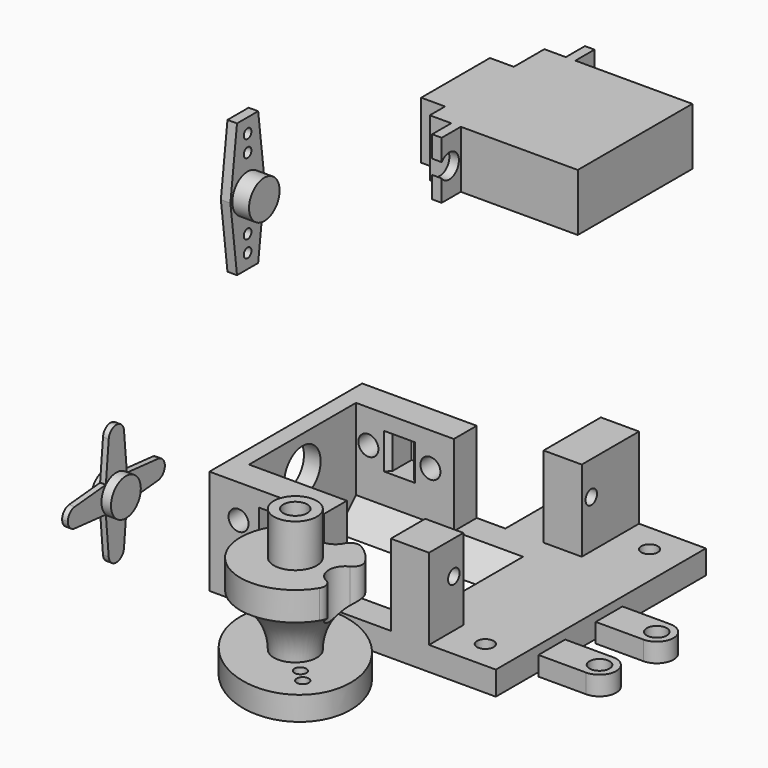
from build123d import *

# Parameters (mm, degrees)
F2_W           = 30
F2_H           = 15
F3_DEPTH       = 5
F5_DEPTH       = 17
F6_R           = 4.75
F7_DEPTH       = 14.501
F8_W           = 4.5
F8_H           = 7.5
F8_R           = 2.1
F9_DEPTH       = 55.001
F10_W          = 30
F10_H          = 12
F11_DEPTH      = 31
F12_W          = 2
F12_H          = 12
F13_DEPTH      = 5
F13_DEPTH_BACK = 35
F14_W          = 18
F14_H          = 12
F15_DEPTH      = 5
F16_R          = 2.75
F17_DEPTH      = 3
F19_DEPTH      = 1.2
F20_COUNT      = 4
F21_R          = 3.9
F22_DEPTH      = 2
F22_DEPTH_BACK = 2.2
F23_R          = 2.5
F24_DEPTH      = 55.501
F25_W          = 8
F25_H          = 9
F25_H_2        = 15
F26_DEPTH      = 17
F28_DEPTH      = 2
F29_R          = 1
F30_DEPTH      = 13.001
F31_R          = 4
F32_DEPTH      = 3.5
F37_R          = 3.5
F38_DEPTH      = 10.6200078449
F39_T1_DEPTH   = 19.8766819715
F41_DEPTH      = 5
F42_R          = 2.5
F43_DEPTH      = 31.0010001
F45_D          = 2.5
F45_DEPTH      = 6
F45_TIP        = 0.7510757738
F46_R          = 2.1
F47_DEPTH      = 4
F49_D          = 3
F49_DEPTH      = 8
F49_TIP        = 0.9012909285
F50_SIZE       = 1
F52_D          = 3.5
F53_R          = 3
F56_DEPTH      = 35


# Not quite as in the source:
# - a fillet or chamfer that OpenCascade refuses, or shapes differently, is made with other operations: its cross-section is extruded or revolved along the edge and cut away or added


with BuildPart() as f3:
    # F2 (on Top) → F3 (new body)
    with BuildSketch(Plane.XY):
        Polygon((0, 15), (0, 0), (60, 0), (60, 40), (30, 40), (0, 40), (0, 25), align=None)
        with Locations((45, 47.5)):
            Rectangle(F2_W, F2_H)
        with BuildLine():
            Line((-6, 15), (0, 15))
            Line((0, 15), (0, 25))
            Line((0, 25), (-6, 25))
            ThreePointArc((-6, 25), (-11, 20), (-6, 15))
        make_face()
    extrude(amount=F3_DEPTH)

    # F4 (on face) → F5 (join)
    with BuildSketch(Plane.XY.offset(5)):
        Polygon((0, 0), (24, 0), (24, 6), (3.5, 6), (3.5, 34), (24, 34), (24, 40), (0, 40), (0, 25), (0, 15), align=None)
    extrude(amount=F5_DEPTH)

    # F6 (on face) → F7 (cut, through all)
    with BuildSketch(Plane.YZ.offset(3.5)):
        with Locations((20, 15)):
            Circle(F6_R)
    extrude(amount=-F7_DEPTH, mode=Mode.SUBTRACT)

    # F8 (on face) → F9 (cut, through all)
    with BuildSketch(Plane.XZ):
        with Locations((12.6, 15)):
            Rectangle(F8_W, F8_H)
        with Locations((6.1, 15)):
            Circle(F8_R)
        with Locations((19.1, 15)):
            Circle(F8_R)
    extrude(amount=-F9_DEPTH, mode=Mode.SUBTRACT)

    # F25 (on face) → F26 (join)
    with BuildSketch(Plane.XY.offset(5)):
        with Locations((42, 4.5)):
            Rectangle(F25_W, F25_H)
        with Locations((42, 47.5)):
            Rectangle(F25_W, F25_H_2)
    extrude(amount=F26_DEPTH)

    # F49
    with Locations(Plane.YZ.offset(46)):
        with Locations((6.5, 15), (42.5, 15)):
            Hole(F49_D / 2, depth=F49_DEPTH)
            with Locations((0, 0, -(F49_DEPTH + F49_TIP / 2))):  # 118° drill point
                Cone(0, F49_D / 2, F49_TIP, mode=Mode.SUBTRACT)

    # F50
    f50_edges = [f3.edges().sort_by_distance(p)[0] for p in [
        (10.35, 34, 15),
        (14.85, 34, 15),
        (10.35, 6, 15),
        (14.85, 6, 15),
    ]]
    chamfer(f50_edges, length=F50_SIZE)

    # F52 (through all)
    with Locations(Plane.XY.offset(5)):
        with Locations((53, 49), (53, 6), (-6, 20)):
            Hole(F52_D / 2)

    # F53
    f53_edges = [f3.edges().sort_by_distance(p)[0] for p in [
        (0, 15, 2.5),
        (0, 25, 2.5),
    ]]
    fillet(f53_edges, radius=F53_R)

    # F55 (on face) → F56 (cut)
    with BuildSketch(Plane.YZ.offset(3.5)):
        Polygon((34, 5), (6, 5), (12, -1), (28, -1), align=None)
    extrude(amount=F56_DEPTH, mode=Mode.SUBTRACT)


with BuildPart() as f11:
    # F10 (on Right) → F11 (new body)
    with BuildSketch(Plane.YZ):
        with Locations((72.7043356746, 58.2544325833)):
            Rectangle(F10_W, F10_H)
    extrude(amount=F11_DEPTH)

    # F12 (on face) → F13 (join, two sides)
    with BuildSketch(Plane.XZ.offset(-57.7043356746)) as f13_sk:
        with Locations((5.5, 58.2544325833)):
            Rectangle(F12_W, F12_H)
    extrude(amount=F13_DEPTH)
    extrude(f13_sk.sketch, amount=-F13_DEPTH_BACK)

    # F14 (on face) → F15 (join)
    with BuildSketch(Plane(origin=(0, 0, 0), x_dir=(0, -1, 0), z_dir=(-1, 0, 0))):
        with Locations((-70.7043356746, 58.2544325833)):
            Rectangle(F14_W, F14_H)
    extrude(amount=F15_DEPTH)

    # F16 (on face) → F17 (join)
    with BuildSketch(Plane(origin=(-5, 0, 0), x_dir=(0, -1, 0), z_dir=(-1, 0, 0))):
        with Locations((-68.2043356746, 58.2544325833)):
            Circle(F16_R)
    extrude(amount=F17_DEPTH)

    # F23 (on face) → F24 (cut, through all)
    with BuildSketch(Plane(origin=(4.5, 0, 0), x_dir=(0, -1, 0), z_dir=(-1, 0, 0))):
        with BuildLine():
            ThreePointArc((-92.7043356746, 56.7544325833), (-89.9137662596, 55.8827243381), (-88.2043356746, 58.2544325833))
            ThreePointArc((-88.2043356746, 58.2544325833), (-89.9137662596, 60.6261408284), (-92.7043356746, 59.7544325833))
            Line((-92.7043356746, 59.7544325833), (-92.7043356746, 56.7544325833))
        make_face()
        with Locations((-54.7043356746, 58.2544325833)):
            Circle(F23_R)
    extrude(amount=-F24_DEPTH, mode=Mode.SUBTRACT)


with BuildPart() as f19:
    # F18 (on Right) → F19 (new body)
    with BuildSketch(Plane.YZ):
        with BuildLine():
            ThreePointArc((-25.8660980829, 41.5474520288), (-27.2194870474, 41.0230042308), (-27.8660980829, 39.7235422843))
            Line((-27.8660980829, 39.7235422843), (-28.6160980829, 31.5974520288))
            Line((-28.6160980829, 31.5974520288), (-36.7421883384, 30.8474520288))
            ThreePointArc((-36.7421883384, 30.8474520288), (-38.041650285, 30.2008409932), (-38.5660980829, 28.8474520288))
            Line((-38.5660980829, 28.8474520288), (-25.8660980829, 28.8474520288))
            Line((-25.8660980829, 28.8474520288), (-25.8660980829, 41.5474520288))
        make_face()
    extrude(amount=F19_DEPTH)

    # F20: F19 ×4 about axis
    f20_axis = Axis((0.6, -25.8660980829, 28.8474520288), (-1, 0, 0))


with BuildPart() as f19_1:
    add(f19.part)
    for i in range(1, F20_COUNT):
        add(f19.part.rotate(f20_axis, i * 360 / F20_COUNT))

    # F21 (on face) → F22 (join, two sides)
    with BuildSketch(Plane.YZ.offset(1.2)) as f22_sk:
        with Locations((-25.8660980829, 28.8474520288)):
            Circle(F21_R)
    extrude(amount=F22_DEPTH)
    extrude(f22_sk.sketch, amount=-F22_DEPTH_BACK)


with BuildPart() as f28:
    # F27 (on Right) → F28 (new body)
    with BuildSketch(Plane.YZ):
        Polygon((4.7284779331, 84.9464619864), (2.9985385872, 70.9464619864), (4.7284779331, 56.9464619864), (10.2685992414, 56.9464619864), (11.9985385872, 70.9464619864), (10.2685992414, 84.9464619864), align=None)
    extrude(amount=F28_DEPTH)

    # F29 (on face) → F30 (cut, through all)
    with BuildSketch(Plane.YZ.offset(2)):
        with Locations((7.4985385872, 78.4464619864)):
            Circle(F29_R)
        with Locations((7.4985385872, 63.4464619864)):
            Circle(F29_R)
        with Locations((7.4985385872, 81.9464619864)):
            Circle(F29_R)
        with Locations((7.4985385872, 59.9464619864)):
            Circle(F29_R)
    extrude(amount=-F30_DEPTH, mode=Mode.SUBTRACT)

    # F31 (on face) → F32 (join)
    with BuildSketch(Plane.YZ.offset(2)):
        with Locations((7.4985385872, 70.9464619864)):
            Circle(F31_R)
    extrude(amount=F32_DEPTH)


with BuildPart() as f36:
    # F35 (on offset) → F36 (revolve)
    with BuildSketch(Plane.XZ.offset(15)):
        with BuildLine():
            Line((30, 31), (30, 0))
            Line((30, 0), (42.5, 0))
            Line((42.5, 0), (42.5, 5))
            Line((42.5, 5), (34.5, 5))
            ThreePointArc((34.5, 5), (36.3983962204, 11.5192024052), (41.5, 16))
            Line((41.5, 16), (41.5, 22))
            Line((41.5, 22), (34.5, 22))
            Line((34.5, 22), (34.5, 31))
            Line((34.5, 31), (30, 31))
        make_face()
    revolve(axis=Axis((30, -15, 15.5), (0, 0, 1)))

    # F37 (on face) → F38 (cut, up to face)
    with BuildSketch(Plane.XY.offset(22)):
        with Locations((30, -4.5)):
            Circle(F37_R)
        with Locations((40.5, -15)):
            Circle(F37_R)
    extrude(amount=-F38_DEPTH, mode=Mode.SUBTRACT)

    # F39: fillet of radius 2 on 4 edges, made by hand

    # F39_s2 → F39_t1 (cut)
    with BuildSketch(Plane.XY.offset(9.0616590143)):
        with BuildLine():
            ThreePointArc((35.9947622921, -5.1860902256), (34.3876430128, -4.9741906463), (33.1513967781, -6.0227272727))
            ThreePointArc((33.1513967781, -6.0227272727), (33.4561100212, -5.052542778), (33.4690688629, -4.0357142857))
            ThreePointArc((33.4690688629, -4.0357142857), (34.7667458746, -4.5344310347), (35.9947622921, -5.1860902256))
        make_face()
        with BuildLine():
            ThreePointArc((26.8486032219, -6.0227272727), (25.6123569872, -4.9741906463), (24.0052377079, -5.1860902256))
            ThreePointArc((24.0052377079, -5.1860902256), (25.2332541254, -4.5344310347), (26.5309311371, -4.0357142857))
            ThreePointArc((26.5309311371, -4.0357142857), (26.5438899788, -5.052542778), (26.8486032219, -6.0227272727))
        make_face()
        with BuildLine():
            ThreePointArc((39.8139097744, -9.0052377079), (40.0258093537, -10.6123569872), (38.9772727273, -11.8486032219))
            ThreePointArc((38.9772727273, -11.8486032219), (39.947457222, -11.5438899788), (40.9642857143, -11.5309311371))
            ThreePointArc((40.9642857143, -11.5309311371), (40.4655689653, -10.2332541254), (39.8139097744, -9.0052377079))
        make_face()
        with BuildLine():
            ThreePointArc((39.8139097744, -20.9947622921), (40.0258093537, -19.3876430128), (38.9772727273, -18.1513967781))
            ThreePointArc((38.9772727273, -18.1513967781), (39.947457222, -18.4561100212), (40.9642857143, -18.4690688629))
            ThreePointArc((40.9642857143, -18.4690688629), (40.4655689653, -19.7667458746), (39.8139097744, -20.9947622921))
        make_face()
    extrude(amount=F39_T1_DEPTH, mode=Mode.SUBTRACT)

    # F40 (on face) → F41 (join, through all)
    with BuildSketch(Plane(origin=(0, 0, 0), x_dir=(1, 0, 0), z_dir=(0, 0, -1))):
        with BuildLine():
            add(Edge.make_bspline(
                [(21.1611652352, 23.8388347648), (1.5652472929, 4.2429168226), (24.6214584113, 0.7826236465), (47.6776695297, -2.6776695297), (44.2173763535, 20.3785415887), (40.7570831774, 43.4347527071), (21.1611652352, 23.8388347648)],
                knots=[4.7123889804, 4.7123889804, 4.7123889804, 6.8067840828, 6.8067840828, 8.9011791852, 8.9011791852, 10.9955742876, 10.9955742876, 10.9955742876], degree=2, weights=[1, 0.5, 1, 0.5, 1, 0.5, 1]))
        make_face()
    extrude(amount=-F41_DEPTH)

    # F42 (on face) → F43 (cut, through all)
    with BuildSketch(Plane.XY.offset(31)):
        with Locations((30, -15)):
            Circle(F42_R)
    extrude(amount=-F43_DEPTH, mode=Mode.SUBTRACT)

    # F45
    with Locations(Plane(origin=(0, 0, 0), x_dir=(1, 0, 0), z_dir=(0, 0, -1))):
        with Locations((22.2218254069, 7.2218254069), (37.7781745931, 22.7781745931), (35.3033008589, 20.3033008589), (24.6966991411, 9.6966991411)):
            Hole(F45_D / 2, depth=F45_DEPTH)
            with Locations((0, 0, -(F45_DEPTH + F45_TIP / 2))):  # 118° drill point
                Cone(0, F45_D / 2, F45_TIP, mode=Mode.SUBTRACT)


with BuildPart() as f47:
    # F46 (on Top) → F47 (new body)
    with BuildSketch(Plane.XY):
        with BuildLine():
            Line((61, 16.9039434447), (61, 9.9039434447))
            Line((61, 9.9039434447), (71, 9.9039434447))
            ThreePointArc((71, 9.9039434447), (74.5, 13.4039434447), (71, 16.9039434447))
            Line((71, 16.9039434447), (61, 16.9039434447))
        make_face()
        with Locations((71, 13.4039434447)):
            Circle(F46_R, mode=Mode.SUBTRACT)
    extrude(amount=F47_DEPTH)


with BuildPart() as f47b:
    # F46 (on Top) → F47, piece 2 (new body)
    with BuildSketch(Plane.XY):
        with BuildLine():
            Line((61, 31.9039434447), (61, 24.9039434447))
            Line((61, 24.9039434447), (71, 24.9039434447))
            ThreePointArc((71, 24.9039434447), (74.5, 28.4039434447), (71, 31.9039434447))
            Line((71, 31.9039434447), (61, 31.9039434447))
        make_face()
        with Locations((71, 28.4039434447)):
            Circle(F46_R, mode=Mode.SUBTRACT)
    extrude(amount=F47_DEPTH)


solid = Compound([f3.part, f11.part, f19_1.part, f28.part, f36.part, f47.part, f47b.part])
